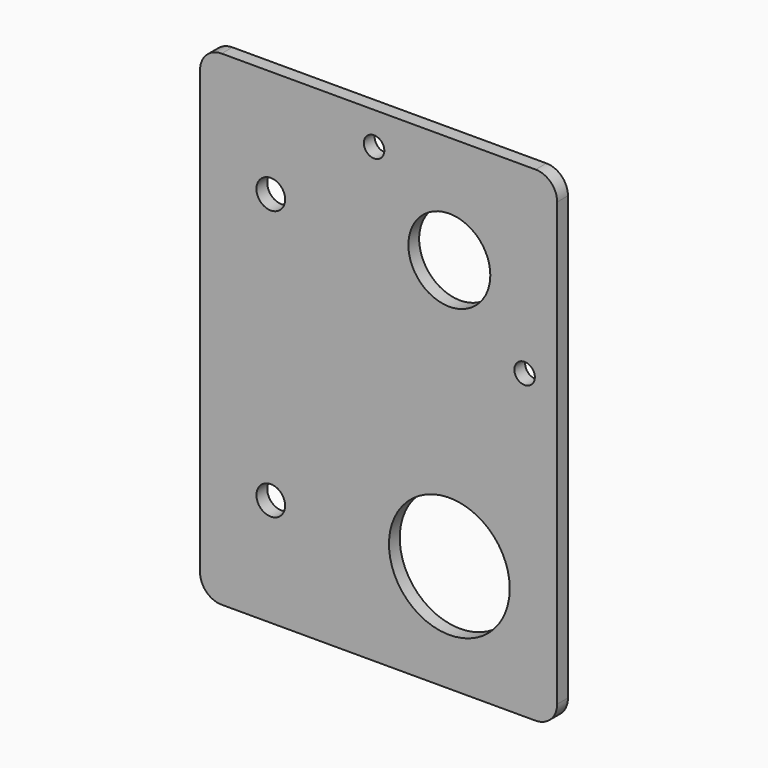
from build123d import *

# Parameters (mm, degrees)
F0_R     = 3.3782
F0_R_2   = 14.224
F0_R_3   = 2.413
F0_R_4   = 9.652
F1_DEPTH = 3.175
F2_R     = 5.08
F3_R     = 5.08


# Not quite as in the source:
# - a length typed as a fraction of an inch, garbled in the dataset ("3 / 203.2 mm" for 3/8 in), is restored


with BuildPart() as f1:
    # F0 (on Front) → F1 (new body)
    with BuildSketch(Plane.XZ):
        Polygon((-25.4, -88.9), (25.4, -88.9), (25.4, 25.4), (-25.4, 25.4), (-58.7248057127, 25.4), (-58.7248057127, -88.9), align=None)
        with Locations((-42.0624028563, -63.5)):
            Circle(F0_R, mode=Mode.SUBTRACT)
        with Locations((0, -63.5)):
            Circle(F0_R_2, mode=Mode.SUBTRACT)
        with Locations((-42.0624028563, 0)):
            Circle(F0_R, mode=Mode.SUBTRACT)
        with Locations((-17.7292, 17.7292)):
            Circle(F0_R_3, mode=Mode.SUBTRACT)
        with Locations((17.7292, -17.7292)):
            Circle(F0_R_3, mode=Mode.SUBTRACT)
        Circle(F0_R_4, mode=Mode.SUBTRACT)
    extrude(amount=F1_DEPTH)

    # F2
    f2_edges = [f1.edges().sort_by_distance(p)[0] for p in [
        (25.4, -1.5875, -88.9),
        (25.4, -1.5875, 25.4),
    ]]
    fillet(f2_edges, radius=F2_R)

    # F3
    f3_edges = [f1.edges().sort_by_distance(p)[0] for p in [
        (-58.724806, -1.5875, 25.4),
        (-58.724806, -1.5875, -88.9),
    ]]
    fillet(f3_edges, radius=F3_R)


solid = f1.part
